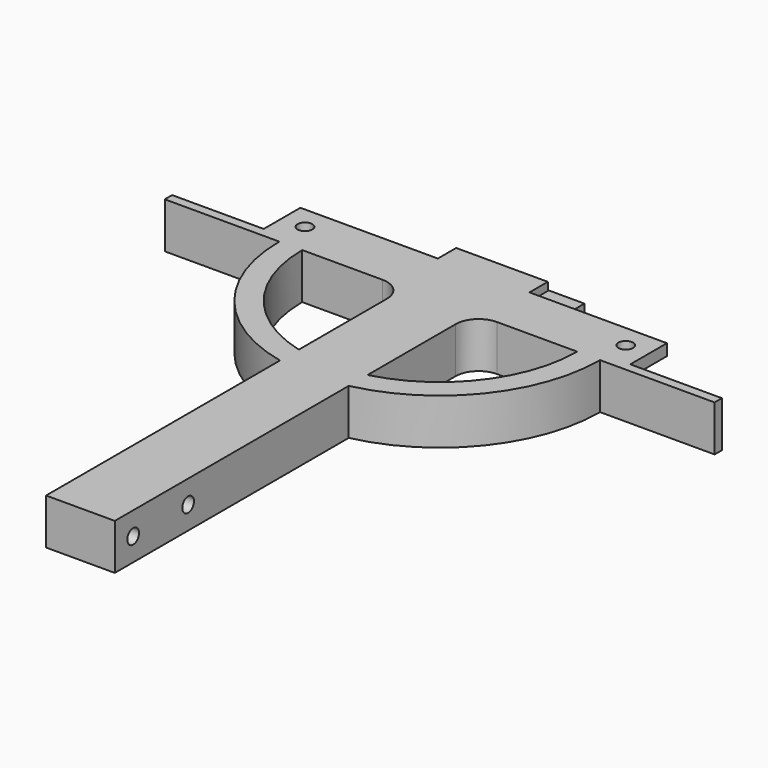
from build123d import *

# Parameters (mm, degrees)
F0_W      = 15
F0_H      = 100
F1_DEPTH  = 5
F2_W      = 80
F2_H      = 10
F3_DEPTH  = 10
F4_W      = 10
F4_H      = 5
F5_DEPTH  = 20
F6_W      = 10
F6_H      = 5
F7_DEPTH  = 20
F8_R      = 1.6
F9_DEPTH  = 10
F10_W     = 67.5
F10_H     = 10
F10_W_2   = 120
F11_DEPTH = 2
F12_R     = 5
F13_R     = 1.6
F14_DEPTH = 15
F15_W     = 20
F15_H     = 10
F16_DEPTH = 5
F17_W     = 20
F17_H     = 6.5
F18_DEPTH = 3
F19_DEPTH = 10
F21_DEPTH = 10


# Not quite as in the source:
# - a pattern or mirror of a feature is missing from the dataset's text; its kind, count and spacing are read off the source's solid


with BuildPart() as f1:
    # F0 (on Top) → F1 (new body, symmetric)
    with BuildSketch(Plane.XY):
        Rectangle(F0_W, F0_H)
    extrude(amount=F1_DEPTH, both=True)

    # F2 (on face) → F3 (join)
    with BuildSketch(Plane(origin=(0, 50, 0), x_dir=(-1, 0, 0), z_dir=(0, 1, 0))):
        Rectangle(F2_W, F2_H)
    extrude(amount=F3_DEPTH)

    # F4 (on face) → F5 (cut)
    with BuildSketch(Plane(origin=(-40, 0, 0), x_dir=(0, -1, 0), z_dir=(-1, 0, 0))):
        with Locations((-55, 0)):
            Rectangle(F4_W, F4_H)
    extrude(amount=-F5_DEPTH, mode=Mode.SUBTRACT)

    # F6 (on face) → F7 (cut)
    with BuildSketch(Plane.YZ.offset(40)):
        with Locations((55, 0)):
            Rectangle(F6_W, F6_H)
    extrude(amount=-F7_DEPTH, mode=Mode.SUBTRACT)

    # F8 (on face) → F9 (cut, through all)
    with BuildSketch(Plane.XY.offset(5)):
        with Locations((-35, 55)):
            Circle(F8_R)
        with Locations((35, 55)):
            Circle(F8_R)
    extrude(amount=-F9_DEPTH, mode=Mode.SUBTRACT)

    # F10 (on face) → F11 (join)
    with BuildSketch(Plane.XZ.offset(-50)):
        with Locations((26.25, 0)):
            Rectangle(F10_W, F10_H)
        Rectangle(F10_W_2, F10_H)
    extrude(amount=F11_DEPTH)

    # F12
    f12_edges = [f1.edges().sort_by_distance(p)[0] for p in [
        (-7.5, 48, 0),
        (7.5, 48, 0),
    ]]
    fillet(f12_edges, radius=F12_R)

    # F13 (on face) → F14 (cut, through all)
    with BuildSketch(Plane(origin=(-7.5, 0, 0), x_dir=(0, -1, 0), z_dir=(-1, 0, 0))):
        with Locations((30, 0)):
            Circle(F13_R)
        with Locations((45, 0)):
            Circle(F13_R)
    extrude(amount=-F14_DEPTH, mode=Mode.SUBTRACT)

    # F15 (on face) → F16 (join)
    with BuildSketch(Plane(origin=(0, 60, 0), x_dir=(-1, 0, 0), z_dir=(0, 1, 0))):
        Rectangle(F15_W, F15_H)
    extrude(amount=F16_DEPTH)

    # F17 (on face) → F18 (cut)
    with BuildSketch(Plane(origin=(0, 65, 0), x_dir=(-1, 0, 0), z_dir=(0, 1, 0))):
        Rectangle(F17_W, F17_H)
    extrude(amount=-F18_DEPTH, mode=Mode.SUBTRACT)

    # F19 (add): a face of the model
    f19_faces = [f1.faces().sort_by_distance(p)[0] for p in [
        (0, 65, -4.125),
    ]]
    extrude(f19_faces, amount=F19_DEPTH)

    # F20 (on face) → F21 (join, through all)
    with BuildSketch(Plane.XY.offset(5)):
        with BuildLine():
            Line((35, 48), (30, 48))
            ThreePointArc((30, 48), (23.7170824513, 29.6288269291), (7.5, 18.9526249034))
            Line((7.5, 18.9526249034), (7.5, 13.8130141721))
            ThreePointArc((7.5, 13.8130141721), (27.2717802866, 26.0625890315), (35, 48))
        make_face()
    f21 = extrude(amount=-F21_DEPTH)

    # F21_copies: F21 across plane
    add(f21.mirror(Plane(origin=(0, 0, 0), x_dir=(0, 0, -1), z_dir=(-1, 0, 0))))


solid = f1.part
